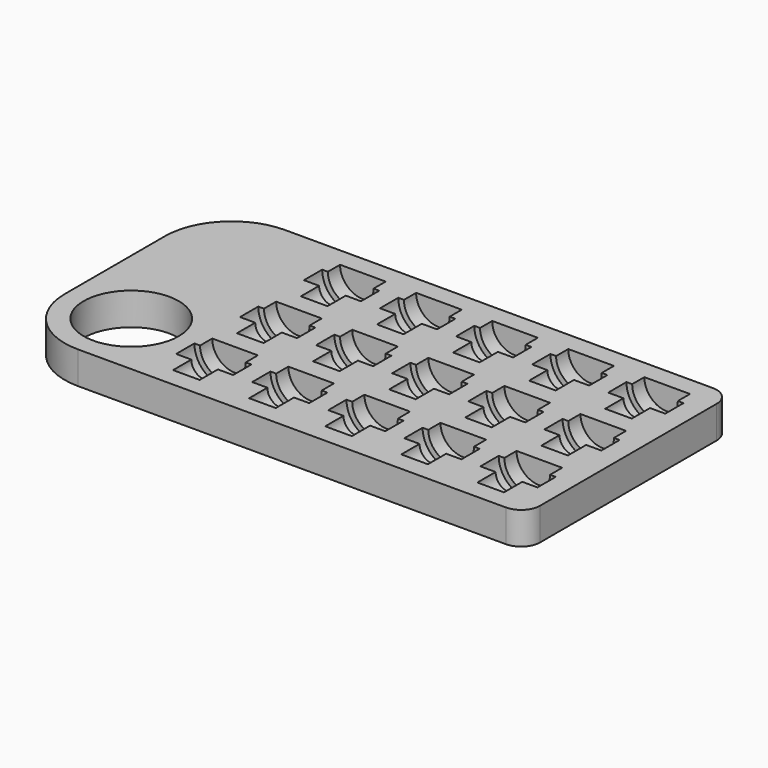
from build123d import *

# Parameters (mm, degrees)
F0_R         = 12.5
F1_DEPTH     = 8.5
F8_TEXT_SIZE = 5.5555555556
F9_DEPTH     = 1


# Not quite as in the source:
# - Text() gives the source's letters only with a copy of the font that has no kerning and outlines rounded to 1/6400 em; it was checked with that copy


with BuildPart() as f1:
    # F0 (on Top) → F1 (new body)
    with BuildSketch(Plane.XY):
        with BuildLine():
            ThreePointArc((0, 17.5), (5.1256313292, 5.1256313292), (17.5, 0))
            Line((17.5, 0), (130, 0))
            ThreePointArc((130, 0), (133.5355339059, 1.4644660941), (135, 5))
            Line((135, 5), (135, 63))
            ThreePointArc((135, 63), (133.5355339059, 66.5355339059), (130, 68))
            Line((130, 68), (17.5, 68))
            ThreePointArc((17.5, 68), (5.1256313292, 62.8743686708), (0, 50.5))
            Line((0, 50.5), (0, 17.5))
        make_face()
        with Locations((17.5, 17.5)):
            Circle(F0_R, mode=Mode.SUBTRACT)
    extrude(amount=F1_DEPTH)

    # F2 (on face) → F3 (revolve, cut)
    with BuildSketch(Plane.XY.offset(8.5)):
        Polygon((48, 21), (42, 21), (42, 17), (42, 11), (42, 5), (45.5, 5), (45.5, 11), (49.5, 11), (49.5, 17), (48, 17), align=None)
        Polygon((48, 42), (42, 42), (42, 38), (42, 32), (42, 26), (45.5, 26), (45.5, 32), (49.5, 32), (49.5, 38), (48, 38), align=None)
        Polygon((48, 63), (42, 63), (42, 59), (42, 53), (42, 47), (45.5, 47), (45.5, 53), (49.5, 53), (49.5, 59), (48, 59), align=None)
    revolve(axis=Axis((42, 50, 8.5), (0, -1, 0)), mode=Mode.SUBTRACT)

    # F2 (on face) → F4 (revolve, cut)
    with BuildSketch(Plane.XY.offset(8.5)):
        Polygon((68, 21), (62, 21), (62, 17), (62, 11), (62, 5), (65.5, 5), (65.5, 11), (69.5, 11), (69.5, 17), (68, 17), align=None)
        Polygon((68, 42), (62, 42), (62, 38), (62, 32), (62, 26), (65.5, 26), (65.5, 32), (69.5, 32), (69.5, 38), (68, 38), align=None)
        Polygon((68, 63), (62, 63), (62, 59), (62, 53), (62, 47), (65.5, 47), (65.5, 53), (69.5, 53), (69.5, 59), (68, 59), align=None)
    revolve(axis=Axis((62, 56, 8.5), (0, -1, 0)), mode=Mode.SUBTRACT)

    # F2 (on face) → F5 (revolve, cut)
    with BuildSketch(Plane.XY.offset(8.5)):
        Polygon((88, 21), (82, 21), (82, 17), (82, 11), (82, 5), (85.5, 5), (85.5, 11), (89.5, 11), (89.5, 17), (88, 17), align=None)
        Polygon((88, 42), (82, 42), (82, 38), (82, 32), (82, 26), (85.5, 26), (85.5, 32), (89.5, 32), (89.5, 38), (88, 38), align=None)
        Polygon((88, 63), (82, 63), (82, 59), (82, 53), (82, 47), (85.5, 47), (85.5, 53), (89.5, 53), (89.5, 59), (88, 59), align=None)
    revolve(axis=Axis((82, 56, 8.5), (0, -1, 0)), mode=Mode.SUBTRACT)

    # F2 (on face) → F6 (revolve, cut)
    with BuildSketch(Plane.XY.offset(8.5)):
        Polygon((108, 21), (102, 21), (102, 17), (102, 11), (102, 5), (105.5, 5), (105.5, 11), (109.5, 11), (109.5, 17), (108, 17), align=None)
        Polygon((108, 42), (102, 42), (102, 38), (102, 32), (102, 26), (105.5, 26), (105.5, 32), (109.5, 32), (109.5, 38), (108, 38), align=None)
        Polygon((108, 63), (102, 63), (102, 59), (102, 53), (102, 47), (105.5, 47), (105.5, 53), (109.5, 53), (109.5, 59), (108, 59), align=None)
    revolve(axis=Axis((102, 56, 8.5), (0, -1, 0)), mode=Mode.SUBTRACT)

    # F2 (on face) → F7 (revolve, cut)
    with BuildSketch(Plane.XY.offset(8.5)):
        Polygon((128, 21), (122, 21), (122, 17), (122, 11), (122, 5), (125.5, 5), (125.5, 11), (129.5, 11), (129.5, 17), (128, 17), align=None)
        Polygon((128, 42), (122, 42), (122, 38), (122, 32), (122, 26), (125.5, 26), (125.5, 32), (129.5, 32), (129.5, 38), (128, 38), align=None)
        Polygon((128, 63), (122, 63), (122, 59), (122, 53), (122, 47), (125.5, 47), (125.5, 53), (129.5, 53), (129.5, 59), (128, 59), align=None)
    revolve(axis=Axis((122, 56, 8.5), (0, -1, 0)), mode=Mode.SUBTRACT)

    # F8 (on face) → F9 (cut)
    with BuildSketch(Plane(origin=(0, 0, 0), x_dir=(1, 0, 0), z_dir=(0, 0, -1))):
        with Locations((30, -9)):
            Text('840', F8_TEXT_SIZE, font='Open Sans', text_align=(TextAlign.LEFT, TextAlign.BOTTOM))
    extrude(amount=-F9_DEPTH, mode=Mode.SUBTRACT)


solid = f1.part
